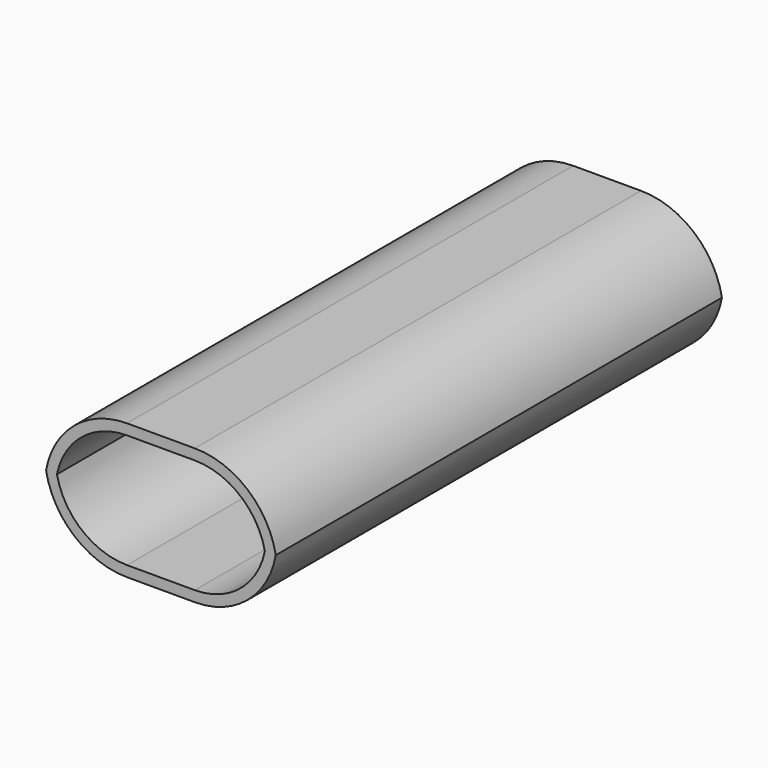
from build123d import *

# Parameters (mm, degrees)
F0_W        = 55.4167628288
F0_H        = 32.3319099844
F1_DEPTH    = 133.096
F2_T1_DEPTH = 231.2096391748
F3_T        = -2.54


# Not quite as in the source:
# - a fillet or chamfer that OpenCascade refuses, or shapes differently, is made with other operations: its cross-section is extruded or revolved along the edge and cut away or added


with BuildPart() as f1:
    # F0 (on Front) → F1 (new body)
    with BuildSketch(Plane.XZ):
        with Locations((-27.7083814144, 16.1659549922)):
            Rectangle(F0_W, F0_H)
    extrude(amount=F1_DEPTH)

    # F2: fillet of radius 19.622727835 on 4 edges, made by hand

    # F2_s2 → F2_t1 (cut)
    with BuildSketch(Plane.XZ.offset(-49.0568195874)):
        with BuildLine():
            ThreePointArc((-35.7940349939, 32.3319099844), (-49.6693989113, 26.5845460669), (-55.4167628288, 12.7091821494))
            Line((-55.4167628288, 12.7091821494), (-55.4167628288, 32.3319099844))
            Line((-55.4167628288, 32.3319099844), (-35.7940349939, 32.3319099844))
        make_face()
        with BuildLine():
            ThreePointArc((0, 12.7091821494), (-5.7473639175, 26.5845460669), (-19.622727835, 32.3319099844))
            Line((-19.622727835, 32.3319099844), (0, 32.3319099844))
            Line((0, 32.3319099844), (0, 12.7091821494))
        make_face()
        with BuildLine():
            ThreePointArc((-19.622727835, 0), (-5.7473639175, 5.7473639175), (0, 19.622727835))
            Line((0, 19.622727835), (0, 0))
            Line((0, 0), (-19.622727835, 0))
        make_face()
        with BuildLine():
            ThreePointArc((-35.7940349939, 0), (-49.6693989113, 5.7473639175), (-55.4167628288, 19.622727835))
            Line((-55.4167628288, 19.622727835), (-55.4167628288, 0))
            Line((-55.4167628288, 0), (-35.7940349939, 0))
        make_face()
    extrude(amount=F2_T1_DEPTH, mode=Mode.SUBTRACT)

    # F3
    f3_openings = [f1.faces().sort_by_distance(p)[0] for p in [
        (-27.708381, -133.096, 16.165955),
    ]]
    offset(amount=F3_T, openings=f3_openings)


solid = f1.part
